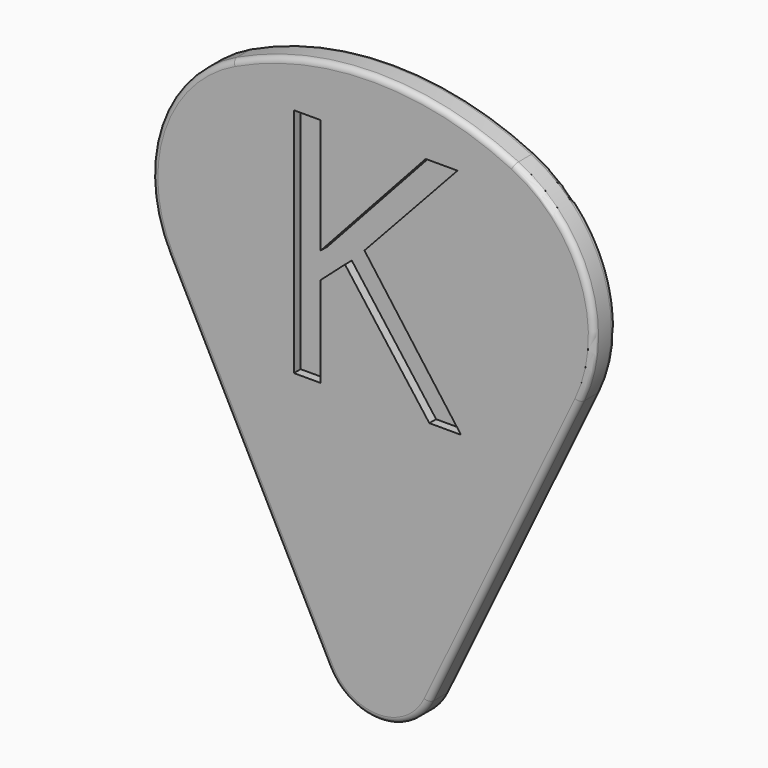
from build123d import *

# Parameters (mm, degrees)
F1_DEPTH     = 1.2192
F2_R         = 0.254
F3_TEXT_SIZE = 14.5469119565
F4_DEPTH     = 0.381


# Not quite as in the source:
# - Text() gives the source's letters only with a copy of the font that has no kerning and outlines rounded to 1/6400 em; it was checked with that copy


with BuildPart() as f1:
    # F0 (on Front) → F1 (new body)
    with BuildSketch(Plane.XZ):
        with BuildLine():
            ThreePointArc((-19.6720034546, 44.0250768827), (-22.9543169758, 40.3238033421), (-22.5848087856, 35.3906023963))
            Line((-22.5848087856, 35.3906023963), (-15.3981215257, 21.4120980362))
            ThreePointArc((-15.3981215257, 21.4120980362), (-13.1058803893, 20.033691746), (-10.8505685538, 21.4717257696))
            Line((-10.8505685538, 21.4717257696), (-4.0859282236, 35.5236255556))
            ThreePointArc((-4.0859282236, 35.5236255556), (-3.8130047195, 40.3729839571), (-7.0471512555, 43.996664452))
            ThreePointArc((-7.0471512555, 43.996664452), (-13.3563449685, 45.447157584), (-19.6720034546, 44.0250768827))
        make_face()
    extrude(amount=F1_DEPTH)

    # F2
    f2_edges = [f1.edges().sort_by_distance(p)[0] for p in [
        (-7.468248, 0, 28.497676),
        (-18.991465, -1.2192, 28.40135),
        (-7.468248, -1.2192, 28.497676),
        (-13.356345, -1.2192, 45.447158),
        (-3.813005, -1.2192, 40.372984),
        (-22.954317, -1.2192, 40.323803),
        (-13.10588, -1.2192, 20.033692),
        (-3.813005, 0, 40.372984),
        (-13.356345, 0, 45.447158),
        (-22.954317, 0, 40.323803),
        (-18.991465, 0, 28.40135),
        (-13.10588, 0, 20.033692),
    ]]
    fillet(f2_edges, radius=F2_R)

    # F3 (on face) → F4 (cut)
    with BuildSketch(Plane.XZ.offset(1.2192)):
        with Locations((-18.3571632668, 32.5386221596)):
            Text('K', F3_TEXT_SIZE, font='Open Sans', text_align=(TextAlign.LEFT, TextAlign.BOTTOM))
    extrude(amount=-F4_DEPTH, mode=Mode.SUBTRACT)


solid = f1.part
